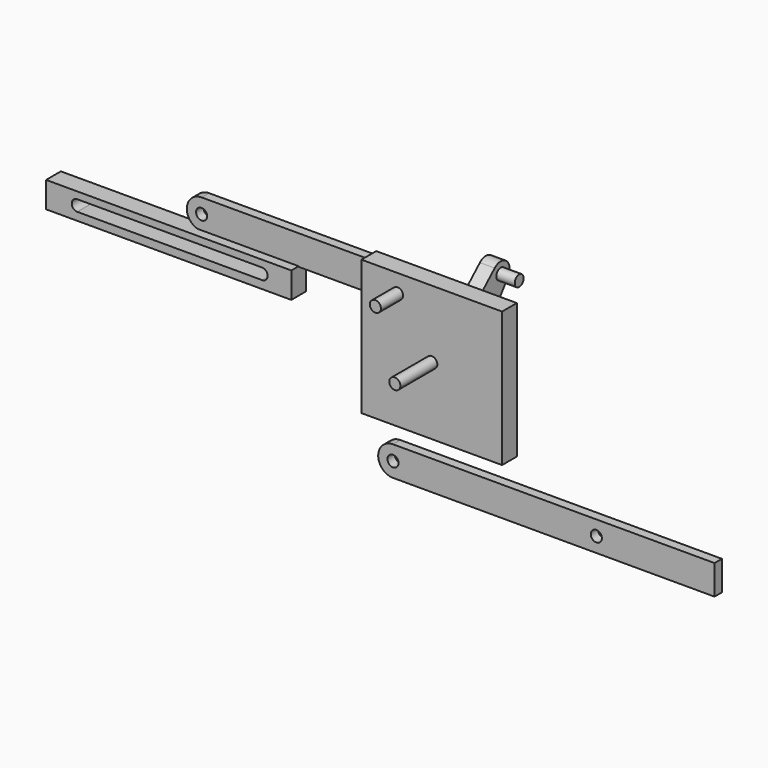
from build123d import *

# Parameters (mm, degrees)
F0_W      = 76.0718137026
F0_H      = 73.10795784
F1_DEPTH  = 10
F2_R      = 3
F3_DEPTH  = 25
F4_R      = 3
F5_DEPTH  = 5
F6_R      = 4
F6_R_2    = 3
F7_DEPTH  = 8
F8_R      = 10
F8_R_2    = 4
F9_DEPTH  = 2
F10_R     = 3
F11_DEPTH = 25
F12_W     = 132.6596662402
F12_H     = 14.0240215696
F13_DEPTH = 10
F14_R     = 3
F15_DEPTH = 10
F18_R     = 3
F19_DEPTH = 5


with BuildPart() as f1:
    # F0 (on Front) → F1 (new body)
    with BuildSketch(Plane.XZ):
        Rectangle(F0_W, F0_H)
    extrude(amount=F1_DEPTH)

    # F2 (on face) → F3 (join)
    with BuildSketch(Plane.XZ.offset(10)):
        Circle(F2_R)
    extrude(amount=F3_DEPTH)


with BuildPart() as f5:
    # F4 (on Front) → F5 (new body)
    with BuildSketch(Plane.XZ):
        with BuildLine():
            Line((-18.4969218779, 34.7494600266), (-128.4969218779, 34.7494600266))
            ThreePointArc((-128.4969218779, 34.7494600266), (-136.4969218779, 26.7494600266), (-128.4969218779, 18.7494600266))
            Line((-128.4969218779, 18.7494600266), (-18.4969218779, 18.7494600266))
            ThreePointArc((-18.4969218779, 18.7494600266), (-10.4969218779, 26.7494600266), (-18.4969218779, 34.7494600266))
        make_face()
        with Locations((-128.4969218779, 26.7494600266)):
            Circle(F4_R, mode=Mode.SUBTRACT)
        with Locations((-18.4969218779, 26.7494600266)):
            Circle(F4_R, mode=Mode.SUBTRACT)
    extrude(amount=F5_DEPTH)


with BuildPart() as f7:
    # F6 (on Right) → F7 (new body)
    with BuildSketch(Plane.YZ):
        with BuildLine():
            Line((22.5574149312, 34.2806509801), (-6.7623428333, 7.3668663219))
            ThreePointArc((-6.7623428333, 7.3668663219), (-6.6537051578, -7.4651327967), (8.0930838649, -5.8738397626))
            Line((8.0930838649, -5.8738397626), (31.4706709501, 26.3362273294))
            ThreePointArc((31.4706709501, 26.3362273294), (30.6070437259, 34.339610865), (22.5574149312, 34.2806509801))
        make_face()
        Circle(F6_R, mode=Mode.SUBTRACT)
        with Locations((26.6148206312, 29.860531187)):
            Circle(F6_R_2, mode=Mode.SUBTRACT)
    extrude(amount=F7_DEPTH)

    # F8 (on face) → F9 (join)
    with BuildSketch(Plane(origin=(0, 0, 0), x_dir=(0, -1, 0), z_dir=(-1, 0, 0))):
        Circle(F8_R)
        Circle(F8_R_2, mode=Mode.SUBTRACT)
    extrude(amount=F9_DEPTH)


with BuildPart() as f11:
    # F10 (on face) → F11 (new body)
    with BuildSketch(Plane(origin=(0, 0, 0), x_dir=(-1, 0, 0), z_dir=(0, 1, 0))):
        with Locations((18.4969218779, 26.7494600266)):
            Circle(F10_R)
    extrude(amount=-F11_DEPTH)


with BuildPart() as f13:
    # F12 (on Front) → F13 (new body)
    with BuildSketch(Plane.XZ):
        with Locations((-142.3116214573, 12.0453021955)):
            Rectangle(F12_W, F12_H)
        with BuildLine():
            ThreePointArc((-191.759181451, 9.3285967857), (-194.759181451, 12.3285967857), (-191.759181451, 15.3285967857))
            Line((-191.759181451, 15.3285967857), (-91.759181451, 15.3285967857))
            ThreePointArc((-91.759181451, 15.3285967857), (-88.759181451, 12.3285967857), (-91.759181451, 9.3285967857))
            Line((-91.759181451, 9.3285967857), (-191.759181451, 9.3285967857))
        make_face(mode=Mode.SUBTRACT)
    extrude(amount=F13_DEPTH)


with BuildPart() as f15:
    # F14 (on face) → F15 (new body)
    with BuildSketch(Plane.YZ.offset(8)):
        with Locations((26.6148206312, 29.860531187)):
            Circle(F14_R)
    extrude(amount=F15_DEPTH)


with BuildPart() as f16_1:
    # F16: copy of F5
    add(f5.part.moved(Location((0, -77, 0))))


with BuildPart() as f19:
    # F18 (on Front) → F19 (new body)
    with BuildSketch(Plane.XZ):
        with BuildLine():
            Line((148.9666812122, -49.1681344882), (-24.9825420976, -49.1681344882))
            ThreePointArc((-24.9825420976, -49.1681344882), (-32.9825420976, -57.1681344882), (-24.9825420976, -65.1681344882))
            Line((-24.9825420976, -65.1681344882), (148.9666812122, -65.1681344882))
            Line((148.9666812122, -65.1681344882), (148.9666812122, -49.1681344882))
        make_face()
        with Locations((-24.9825420976, -57.1681344882)):
            Circle(F18_R, mode=Mode.SUBTRACT)
        with Locations((85.0174579024, -57.1681344882)):
            Circle(F18_R, mode=Mode.SUBTRACT)
    extrude(amount=F19_DEPTH)


solid = Compound([f1.part, f5.part, f7.part, f11.part, f13.part, f15.part, f19.part])
